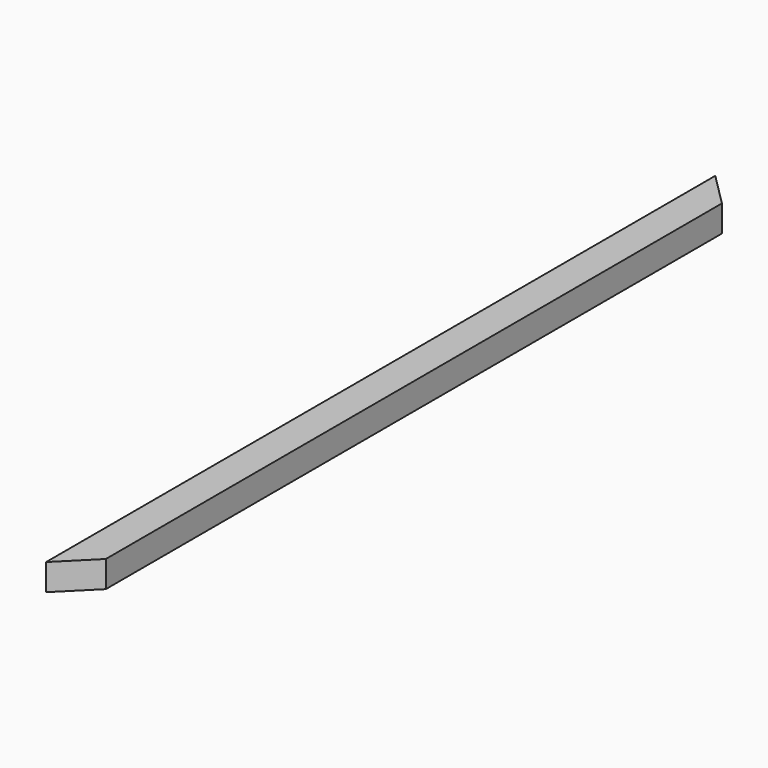
from build123d import *

# Parameters (mm, degrees)
F0_W     = 50
F0_H     = 40
F1_DEPTH = 1260
F2_SIZE2 = 49.99999
F2_SIZE  = 49.99999


# Not quite as in the source:
# - a fillet or chamfer is up to 0.001 mm smaller than in the source, because OpenCascade refuses the exact size


with BuildPart() as f1:
    # F0 (on Front) → F1 (new body)
    with BuildSketch(Plane.XZ):
        with Locations((25, 20)):
            Rectangle(F0_W, F0_H)
    extrude(amount=F1_DEPTH)

    # F2 (size 50 and 50 in the source; OpenCascade refuses exactly that, so slightly less here)
    f2_edges = [f1.edges().sort_by_distance(p)[0] for p in [
        (50, 0, 20),
        (50, -1260, 20),
    ]]
    chamfer(f2_edges, length=F2_SIZE, length2=F2_SIZE2)


solid = f1.part
